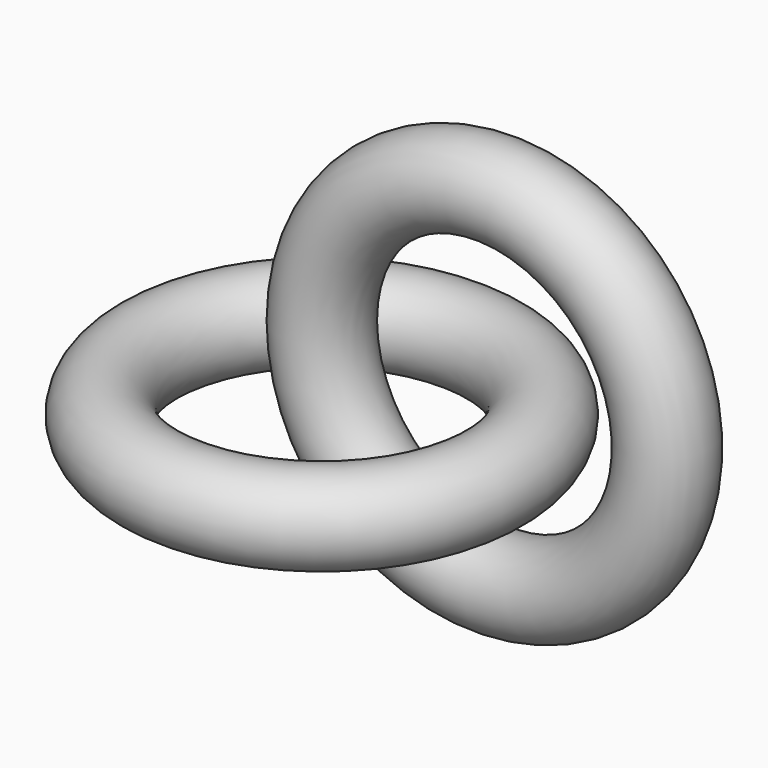
from build123d import *

# Parameters (mm, degrees)
F0_R = 12.5
F2_R = 12.5


# Not quite as in the source:
# - a feature names something its author has since deleted; it is built from what else it names


with BuildPart() as f1:
    # F0 (on Front) → F1 (revolve)
    with BuildSketch(Plane.XZ):
        with Locations((-50, -24)):
            Circle(F0_R)
    revolve(axis=Axis((0, 0, -0.2122972161), (0, 0, -1)))


with BuildPart() as f3:
    # F2 (on Top) → F3 (revolve)
    with BuildSketch(Plane.XY):
        Circle(F2_R)
    revolve(axis=Axis((50, -5.6015, 0), (0, -1, 0)))


solid = Compound([f1.part, f3.part])
